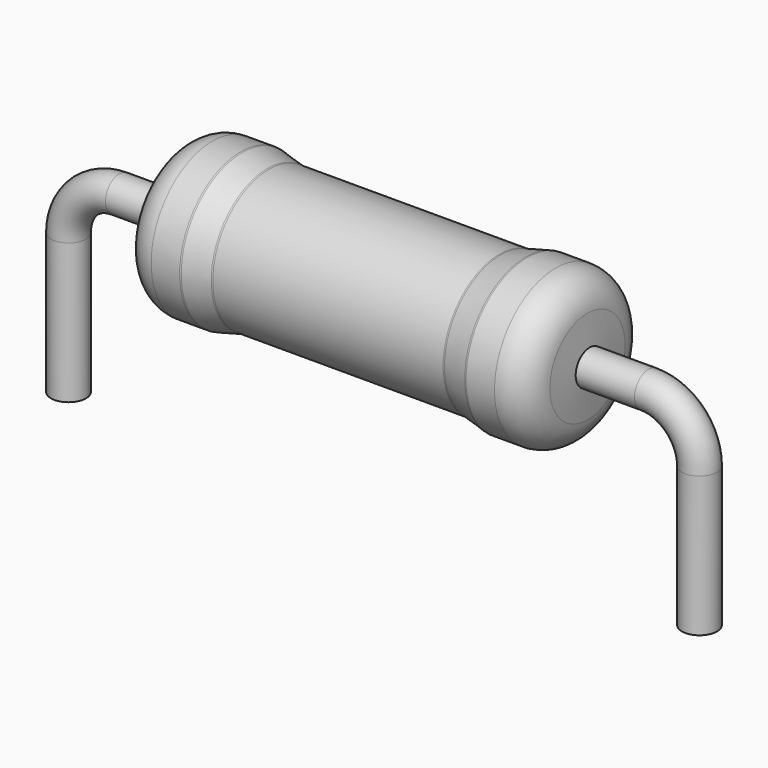
from build123d import *

# Parameters (mm, degrees)
F3_R = 0.275


with BuildPart() as f1:
    # F0 (on Top) → F1 (revolve)
    with BuildSketch(Plane.XY):
        with BuildLine():
            Line((-3.1939512269, 0.7378709646), (-3.25, 0))
            Line((-3.25, 0), (0, 0))
            Line((0, 0), (0, 1.1))
            Line((0, 1.1), (-1.8078035141, 1.1))
            ThreePointArc((-1.8078035141, 1.1), (-1.8195402238, 1.1006911401), (-1.8311146993, 1.1027550071))
            Line((-1.8311146993, 1.1027550071), (-2.2252893382, 1.1972449929))
            ThreePointArc((-2.2252893382, 1.1972449929), (-2.2368638136, 1.1993088599), (-2.2486005233, 1.2))
            Line((-2.2486005233, 1.2), (-2.6953874998, 1.2))
            ThreePointArc((-2.6953874998, 1.2), (-3.0352878658, 1.0666984335), (-3.1939512269, 0.7378709646))
        make_face()
    revolve(axis=Axis((-1.625, 0, 0), (-1, 0, 0)))

    # F2: F1 across face


with BuildPart() as f1_1:
    add(f1.part)
    add(f1.part.mirror(Plane.YZ))


with BuildPart() as f5:
    # F5: sweep along a path in F4
    with BuildLine(Plane.XZ) as f5_path:
        Line((0, 0), (4.153, 0))
        ThreePointArc((4.153, 0), (4.7186854249, -0.2343145751), (4.953, -0.8))
        Line((4.953, -0.8), (4.953, -3))
    # F3 (on Right) → F5 (sweep)
    with BuildSketch(Plane.YZ):
        Circle(F3_R)
    sweep(path=f5_path.line)

    # F6: F5 across plane


with BuildPart() as f5_1:
    add(f5.part)
    add(f5.part.mirror(Plane.YZ))


solid = Compound([f1_1.part, f5_1.part])
